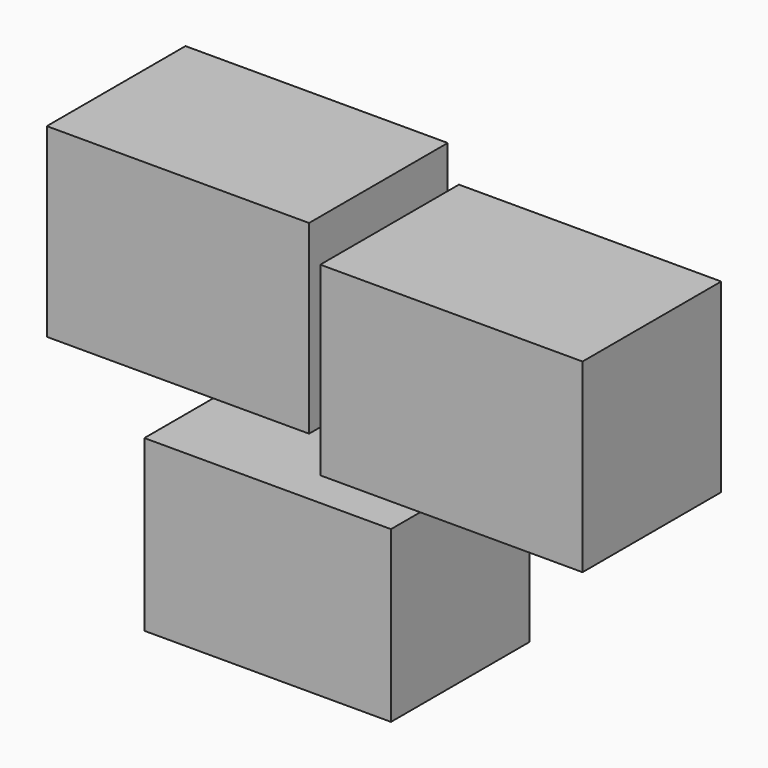
from build123d import *

# Parameters (mm, degrees)
F0_W     = 134.5095438883
F0_H     = 95.1358787715
F1_DEPTH = 88.9
F4_W     = 126.4854110777
F4_H     = 87.0437249541
F5_DEPTH = 88.9
F6_W     = 75.1584813697
F6_H     = 0.2573542297
F7_DEPTH = 0.254


# Not quite as in the source:
# - a feature names something its author has since deleted; it is built from what else it names


with BuildPart() as f1:
    # F0 (on Front) → F1 (new body)
    with BuildSketch(Plane.XZ):
        with Locations((-80.2886434831, -2.5838185102)):
            Rectangle(F0_W, F0_H)
    extrude(amount=F1_DEPTH)


with BuildPart() as f2_1:
    # F2: instance of F1
    add(f1.part.mirror(Plane.YZ))


with BuildPart() as f1_1:
    # F3: moved
    add(f1.part.moved(Location((0, 25.4, 0))))


with BuildPart() as f5:
    # F4 (on Front) → F5 (new body)
    with BuildSketch(Plane.XZ):
        with Locations((-13.9376055449, -106.1658747494)):
            Rectangle(F4_W, F4_H)
    extrude(amount=F5_DEPTH)


with BuildPart() as f7:
    # F6 (on Front) → F7 (new body)
    with BuildSketch(Plane.XZ):
        with Locations((-38.7289650389, -58.4174264222)):
            Rectangle(F6_W, F6_H)
    extrude(amount=F7_DEPTH)


solid = Compound([f2_1.part, f1_1.part, f5.part, f7.part])
